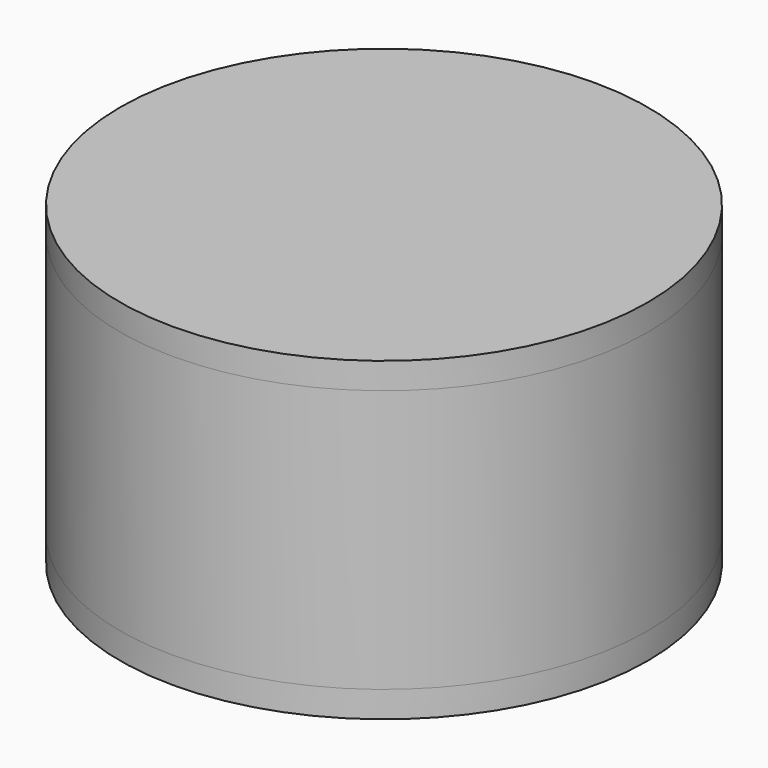
from build123d import *

# Parameters (mm, degrees)
F0_R     = 25.5
F1_DEPTH = 25.4
F2_DEPTH = 2.54
F3_DEPTH = 2.54


with BuildPart() as f1:
    # F0 (on Top) → F1 (new body)
    with BuildSketch(Plane.XY):
        Circle(F0_R)
    extrude(amount=F1_DEPTH)


with BuildPart() as f2:
    # F2 (new): a face of the model
    f2_faces = [f1.part.faces().sort_by_distance(p)[0] for p in [
        (0, 0, 0),
    ]]
    extrude(f2_faces, amount=F2_DEPTH)


with BuildPart() as f3:
    # F3 (new): a face of the model
    f3_faces = [f1.part.faces().sort_by_distance(p)[0] for p in [
        (0, 0, 25.4),
    ]]
    extrude(f3_faces, amount=F3_DEPTH)


solid = Compound([f1.part, f2.part, f3.part])
